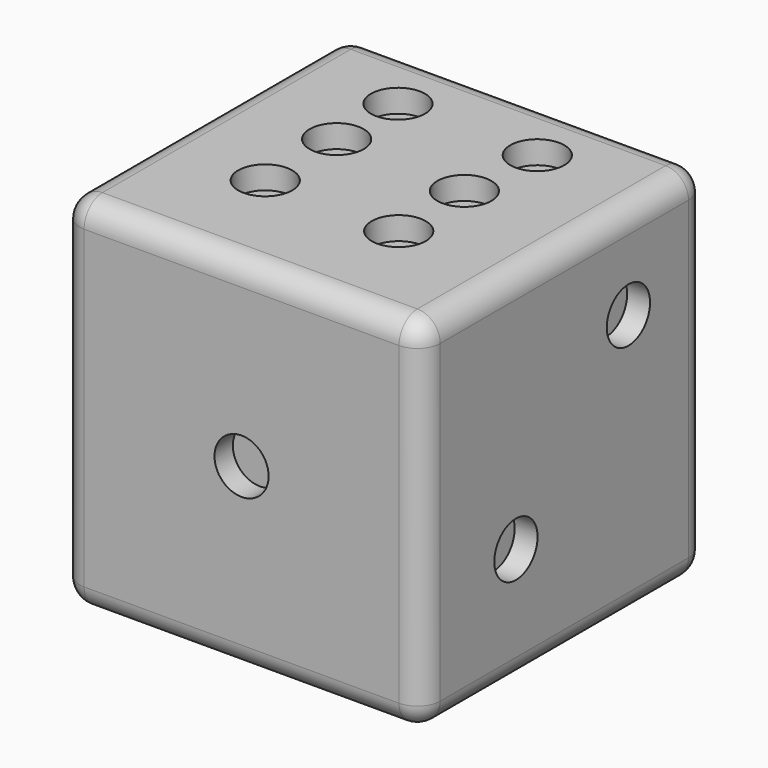
from build123d import *

# Parameters (mm, degrees)
F0_W      = 200
F0_H      = 200
F1_DEPTH  = 197.4596
F2_R      = 12.7
F3_R      = 15
F4_DEPTH  = 12.7
F6_R      = 15
F7_DEPTH  = 12.7
F5_R      = 15
F8_DEPTH  = 12.7
F9_R      = 15
F10_DEPTH = 12.7
F11_R     = 15
F12_DEPTH = 12.7
F13_R     = 15
F14_DEPTH = 12.7


# Not quite as in the source:
# - a feature names something its author has since deleted; it is built from what else it names


with BuildPart() as f1:
    # F0 (on Front) → F1 (new body)
    with BuildSketch(Plane.XZ):
        Rectangle(F0_W, F0_H)
    extrude(amount=F1_DEPTH)

    # F2
    f2_edges = [f1.edges().sort_by_distance(p)[0] for p in [
        (100, -98.7298, -100),
        (100, -98.7298, 100),
        (100, 0, 0),
        (100, -197.4596, 0),
        (-100, -98.7298, 100),
        (0, 0, 100),
        (0, -197.4596, 100),
        (0, 0, -100),
        (-100, 0, 0),
        (-100, -98.7298, -100),
        (0, -197.4596, -100),
        (-100, -197.4596, 0),
    ]]
    fillet(f2_edges, radius=F2_R)

    # F3 (on face) → F4 (cut)
    with BuildSketch(Plane.XZ.offset(197.4596)):
        Circle(F3_R)
    extrude(amount=-F4_DEPTH, mode=Mode.SUBTRACT)

    # F6 (on face) → F7 (cut)
    with BuildSketch(Plane(origin=(0, 0, 0), x_dir=(-1, 0, 0), z_dir=(0, 1, 0))):
        with Locations((54.645486176, 53.4084625542)):
            Circle(F6_R)
        Circle(F6_R)
        with Locations((-55.5655397475, -50.3540486097)):
            Circle(F6_R)
    extrude(amount=-F7_DEPTH, mode=Mode.SUBTRACT)

    # F5 (on face) → F8 (cut)
    with BuildSketch(Plane.YZ.offset(100)):
        with Locations((-132.281050086, -34.5258712769)):
            Circle(F5_R)
        with Locations((-54.3126091361, 48.1324009597)):
            Circle(F5_R)
    extrude(amount=-F8_DEPTH, mode=Mode.SUBTRACT)

    # F9 (on face) → F10 (cut)
    with BuildSketch(Plane(origin=(-100, 0, 0), x_dir=(0, -1, 0), z_dir=(-1, 0, 0))):
        with Locations((42.3903614283, 50.2816922963)):
            Circle(F9_R)
        with Locations((39.9255715311, -43.3802828193)):
            Circle(F9_R)
        with Locations((148.3762711287, 55.2112646401)):
            Circle(F9_R)
        with Locations((153.7988185883, -42.8873226047)):
            Circle(F9_R)
    extrude(amount=-F10_DEPTH, mode=Mode.SUBTRACT)

    # F11 (on face) → F12 (cut)
    with BuildSketch(Plane(origin=(0, 0, -100), x_dir=(1, 0, 0), z_dir=(0, 0, -1))):
        with Locations((0, 105.1476597786)):
            Circle(F11_R)
        with Locations((53.2865412533, 56.5827190876)):
            Circle(F11_R)
        with Locations((-45.8668917418, 53.8846664131)):
            Circle(F11_R)
        with Locations((-53.9610497653, 157.759681344)):
            Circle(F11_R)
        with Locations((59.3571513891, 154.3871164322)):
            Circle(F11_R)
    extrude(amount=-F12_DEPTH, mode=Mode.SUBTRACT)

    # F13 (on face) → F14 (cut)
    with BuildSketch(Plane.XY.offset(100)):
        with Locations((-39.4590161741, -39.7198908031)):
            Circle(F13_R)
        with Locations((37.8009901579, -39.7198908031)):
            Circle(F13_R)
        with Locations((-39.4590161741, -82.2142139077)):
            Circle(F13_R)
        with Locations((34.062910825, -85.5867788196)):
            Circle(F13_R)
        with Locations((-39.4590161741, -131.7378137109)):
            Circle(F13_R)
        with Locations((35.4119352996, -132.8026950359)):
            Circle(F13_R)
    extrude(amount=-F14_DEPTH, mode=Mode.SUBTRACT)


solid = f1.part
